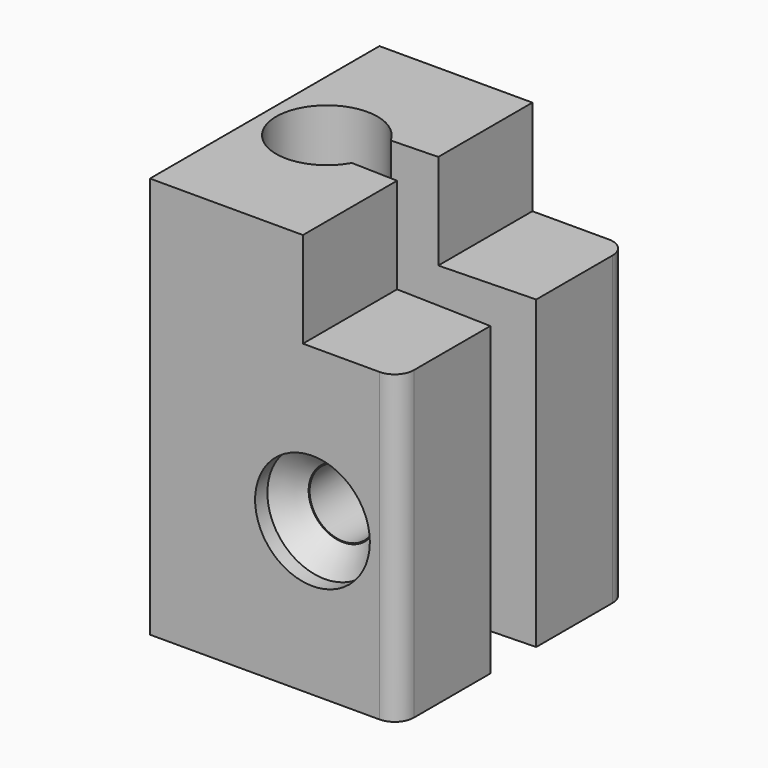
from build123d import *

# Parameters (mm, degrees)
F0_W      = 13
F0_H      = 15
F1_DEPTH  = 21
F3_DEPTH  = 21
F4_W      = 5
F4_H      = 15
F5_DEPTH  = 5
F6_R      = 1.75
F7_DEPTH  = 42
F8_R      = 1.75
F9_DEPTH  = 2
F10_R     = 3
F10_R_2   = 1.75
F11_DEPTH = 2
F12_SIZE  = 1.2
F13_R     = 1


# Not quite as in the source:
# - an extrude ends at something that could not be found from the text; its depth is read off the source's solid


with BuildPart() as f1:
    # F0 (on Top) → F1 (new body)
    with BuildSketch(Plane.XY):
        Rectangle(F0_W, F0_H)
    extrude(amount=F1_DEPTH)

    # F2 (on face) → F3 (cut, through all)
    with BuildSketch(Plane.XY.offset(21)):
        with BuildLine():
            ThreePointArc((-0.9255449651, -1.272559936), (-0.682675922, -0.6567701872), (-0.6, 0))
            ThreePointArc((-0.6, 0), (-0.682675922, 0.6567701872), (-0.9255449651, 1.272559936))
            Line((-0.9255449651, 1.272559936), (-0.9255449651, -1.272559936))
        make_face()
        with BuildLine():
            ThreePointArc((-0.9255449651, 1.272559936), (-0.682675922, 0.6567701872), (-0.6, 0))
            ThreePointArc((-0.6, 0), (-0.682675922, -0.6567701872), (-0.9255449651, -1.272559936))
            Line((-0.9255449651, -1.272559936), (6.5, -1.5))
            Line((6.5, -1.5), (6.5, 1.5))
            Line((6.5, 1.5), (-0.9255449651, 1.272559936))
        make_face()
        with BuildLine():
            Line((-0.9255449651, -1.272559936), (-0.9255449651, 1.272559936))
            ThreePointArc((-0.9255449651, 1.272559936), (-5.9, 0), (-0.9255449651, -1.272559936))
        make_face()
    extrude(amount=-F3_DEPTH, mode=Mode.SUBTRACT)

    # F4 (on face) → F5 (cut)
    with BuildSketch(Plane.XY.offset(21)):
        with Locations((4, 0)):
            Rectangle(F4_W, F4_H)
    extrude(amount=-F5_DEPTH, mode=Mode.SUBTRACT)

    # F6 (on face) → F7 (cut, through all)
    with BuildSketch(Plane.XZ.offset(7.5)):
        with Locations((2, 8)):
            Circle(F6_R)
    extrude(amount=-F7_DEPTH, mode=Mode.SUBTRACT)

    # F8 (on face) → F9 (cut)
    with BuildSketch(Plane(origin=(0, 7.5, 0), x_dir=(-1, 0, 0), z_dir=(0, 1, 0))):
        Polygon((-0.2679491924, 11), (-3.7320508076, 11), (-5.4641016151, 8), (-3.7320508076, 5), (-0.2679491924, 5), (1.4641016151, 8), align=None)
        with Locations((-2, 8)):
            Circle(F8_R, mode=Mode.SUBTRACT)
    extrude(amount=-F9_DEPTH, mode=Mode.SUBTRACT)

    # F10 (on face) → F11 (cut)
    with BuildSketch(Plane.XZ.offset(7.5)):
        with Locations((2, 8)):
            Circle(F10_R)
        with Locations((2, 8)):
            Circle(F10_R_2, mode=Mode.SUBTRACT)
    extrude(amount=-F11_DEPTH, mode=Mode.SUBTRACT)

    # F12
    f12_edges = [f1.edges().sort_by_distance(p)[0] for p in [
        (-1, -5.5, 8),
    ]]
    chamfer(f12_edges, length=F12_SIZE)

    # F13
    f13_edges = [f1.edges().sort_by_distance(p)[0] for p in [
        (6.5, -7.5, 8),
        (6.5, 7.5, 8),
    ]]
    fillet(f13_edges, radius=F13_R)


solid = f1.part
